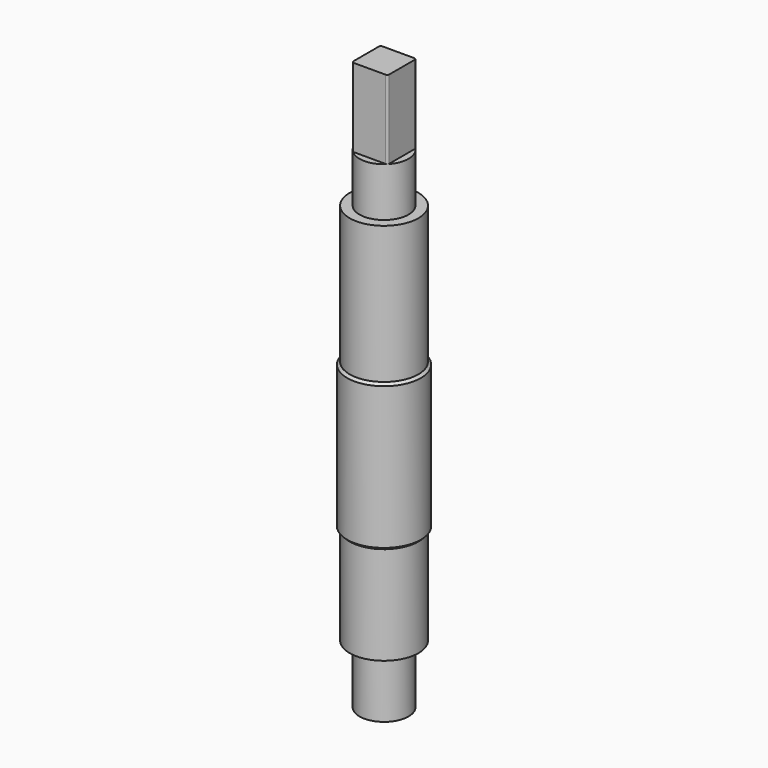
from build123d import *

# Parameters (mm, degrees)
F0_R      = 3.5
F1_DEPTH  = 14
F2_R      = 2.5
F3_DEPTH  = 5
F5_DEPTH  = 8
F6_R      = 3.75
F7_DEPTH  = 15
F8_R      = 3.5
F9_DEPTH  = 10
F10_SIZE  = 0.24999
F11_R     = 2.5
F12_DEPTH = 6


# Not quite as in the source:
# - a fillet or chamfer is up to 0.001 mm smaller than in the source, because OpenCascade refuses the exact size


with BuildPart() as f1:
    # F0 (on Top) → F1 (new body)
    with BuildSketch(Plane.XY):
        Circle(F0_R)
    extrude(amount=F1_DEPTH)

    # F2 (on face) → F3 (join)
    with BuildSketch(Plane.XY.offset(14)):
        Circle(F2_R)
    extrude(amount=F3_DEPTH)

    # F4 (on face) → F5 (join)
    with BuildSketch(Plane.XY.offset(19)):
        with BuildLine():
            ThreePointArc((1.8263455967, 1.6263455967), (1.767766953, 1.767766953), (1.6263455967, 1.8263455967))
            Line((1.6263455967, 1.8263455967), (-1.6263455967, 1.8263455967))
            ThreePointArc((-1.6263455967, 1.8263455967), (-1.767766953, 1.767766953), (-1.8263455967, 1.6263455967))
            Line((-1.8263455967, 1.6263455967), (-1.8263455967, -1.6263455967))
            ThreePointArc((-1.8263455967, -1.6263455967), (-1.767766953, -1.767766953), (-1.6263455967, -1.8263455967))
            Line((-1.6263455967, -1.8263455967), (1.6263455967, -1.8263455967))
            ThreePointArc((1.6263455967, -1.8263455967), (1.767766953, -1.767766953), (1.8263455967, -1.6263455967))
            Line((1.8263455967, -1.6263455967), (1.8263455967, 1.6263455967))
        make_face()
    extrude(amount=F5_DEPTH)

    # F6 (on face) → F7 (join)
    with BuildSketch(Plane(origin=(0, 0, 0), x_dir=(1, 0, 0), z_dir=(0, 0, -1))):
        Circle(F6_R)
    extrude(amount=F7_DEPTH)

    # F8 (on face) → F9 (join)
    with BuildSketch(Plane(origin=(0, 0, -15), x_dir=(1, 0, 0), z_dir=(0, 0, -1))):
        Circle(F8_R)
    extrude(amount=F9_DEPTH)

    # F10 (size 0.25 in the source; OpenCascade refuses exactly that, so slightly less here)
    f10_edges = [f1.edges().sort_by_distance(p)[0] for p in [
        (-3.75, 0, 0),
        (-3.75, 0, -15),
    ]]
    chamfer(f10_edges, length=F10_SIZE)

    # F11 (on face) → F12 (join)
    with BuildSketch(Plane(origin=(0, 0, -25), x_dir=(1, 0, 0), z_dir=(0, 0, -1))):
        Circle(F11_R)
    extrude(amount=F12_DEPTH)


solid = f1.part
